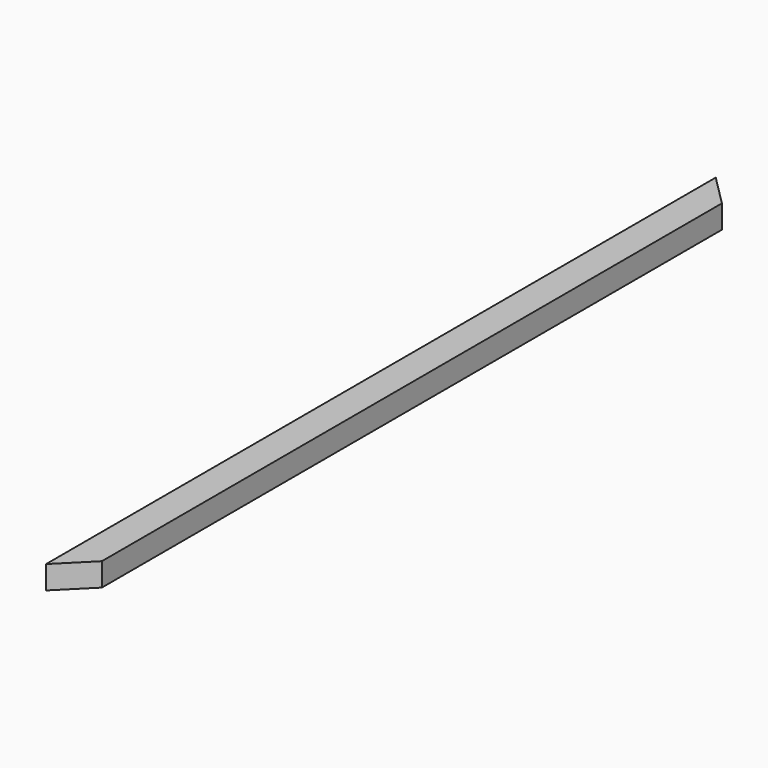
from build123d import *

# Parameters (mm, degrees)
F0_W     = 25.4
F0_H     = 685.8
F1_DEPTH = 19.05
F2_SIZE  = 25.39999


# Not quite as in the source:
# - a fillet or chamfer is up to 0.001 mm smaller than in the source, because OpenCascade refuses the exact size


with BuildPart() as f1:
    # F0 (on Top) → F1 (new body)
    with BuildSketch(Plane.XY):
        with Locations((-3.6795400083, 309.0868617729)):
            Rectangle(F0_W, F0_H)
    extrude(amount=F1_DEPTH)

    # F2 (size 25.4 in the source; OpenCascade refuses exactly that, so slightly less here)
    f2_edges = [f1.edges().sort_by_distance(p)[0] for p in [
        (9.02046, -33.813138, 9.525),
        (9.02046, 651.986862, 9.525),
    ]]
    chamfer(f2_edges, length=F2_SIZE)


solid = f1.part
